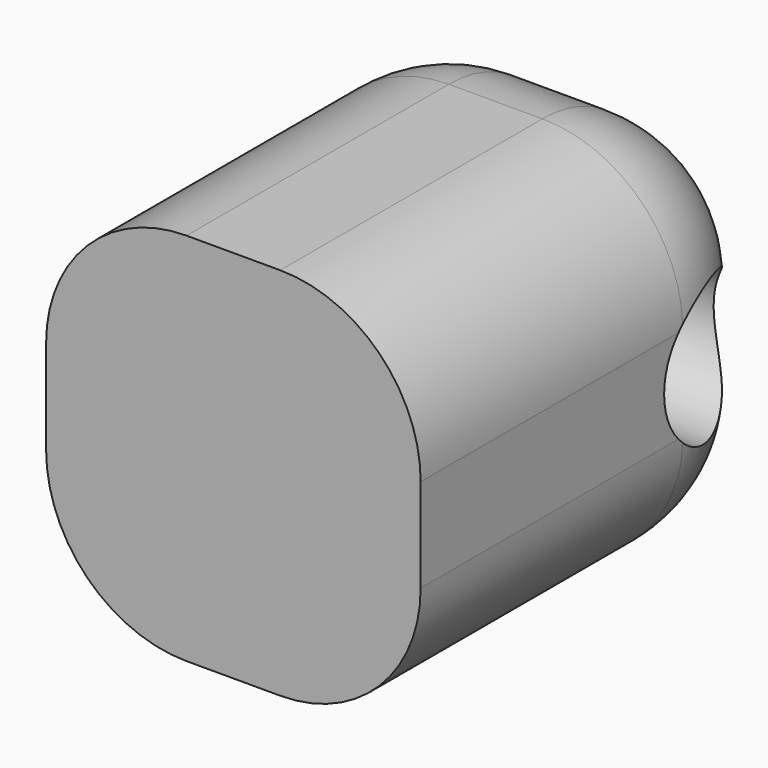
from build123d import *

# Parameters (mm, degrees)
F0_W         = 20
F0_H         = 20
F1_DEPTH     = 25
F2_R         = 3.75
F3_DEPTH     = 25
F4_R         = 7.5
F5_T1_DEPTH  = 36.25
F5_T3_DEPTH  = 5
F5_T6_ANGLE  = 90
F5_T8_ANGLE  = 90
F5_T10_ANGLE = 90
F5_T12_ANGLE = 90


# Not quite as in the source:
# - a fillet or chamfer that OpenCascade refuses, or shapes differently, is made with other operations: its cross-section is extruded or revolved along the edge and cut away or added


with BuildPart() as f1:
    # F0 (on Front) → F1 (new body)
    with BuildSketch(Plane.XZ):
        Rectangle(F0_W, F0_H)
    extrude(amount=F1_DEPTH)

    # F2 (on Right) → F3 (cut, symmetric)
    with BuildSketch(Plane.YZ):
        with Locations((-5, 0)):
            Circle(F2_R)
    extrude(amount=F3_DEPTH, both=True, mode=Mode.SUBTRACT)

    # F4
    f4_edges = [f1.edges().sort_by_distance(p)[0] for p in [
        (0, 0, 10),
        (0, 0, -10),
    ]]
    fillet(f4_edges, radius=F4_R)

    # F5: fillet of radius 7.5 on 8 edges, made by hand

    # F5_s2 → F5_t1 (cut)
    with BuildSketch(Plane.XZ.offset(7.5)):
        with BuildLine():
            ThreePointArc((-10, 2.5), (-7.8033008589, 7.8033008589), (-2.5, 10))
            Line((-2.5, 10), (-10, 10))
            Line((-10, 10), (-10, 2.5))
        make_face()
        with BuildLine():
            ThreePointArc((10, 2.5), (7.8033008589, 7.8033008589), (2.5, 10))
            Line((2.5, 10), (10, 10))
            Line((10, 10), (10, 2.5))
        make_face()
        with BuildLine():
            ThreePointArc((-2.5, -10), (-7.8033008589, -7.8033008589), (-10, -2.5))
            Line((-10, -2.5), (-10, -10))
            Line((-10, -10), (-2.5, -10))
        make_face()
        with BuildLine():
            ThreePointArc((2.5, -10), (7.8033008589, -7.8033008589), (10, -2.5))
            Line((10, -2.5), (10, -10))
            Line((10, -10), (2.5, -10))
        make_face()
    extrude(amount=F5_T1_DEPTH, mode=Mode.SUBTRACT)

    # F5_s4 → F5_t3 (cut)
    with BuildSketch(Plane.XY.offset(-2.5)):
        with BuildLine():
            ThreePointArc((10, -7.5), (7.8033008589, -2.1966991411), (2.5, 0))
            Line((2.5, 0), (10, 0))
            Line((10, 0), (10, -7.5))
        make_face()
        with BuildLine():
            ThreePointArc((-10, -7.5), (-7.8033008589, -2.1966991411), (-2.5, 0))
            Line((-2.5, 0), (-10, 0))
            Line((-10, 0), (-10, -7.5))
        make_face()
    extrude(amount=F5_T3_DEPTH, mode=Mode.SUBTRACT)

    # F5_s5 → F5_t6 (revolve, cut)
    with BuildSketch(Plane.XY.offset(2.5)):
        with BuildLine():
            ThreePointArc((-10, -7.5), (-7.8033008589, -2.1966991411), (-2.5, 0))
            Line((-2.5, 0), (-10, 0))
            Line((-10, 0), (-10, -7.5))
        make_face()
    revolve(axis=Axis((-10, -7.5, 2.5), (1, 0, 0)), revolution_arc=F5_T6_ANGLE, mode=Mode.SUBTRACT)

    # F5_s7 → F5_t8 (revolve, cut)
    with BuildSketch(Plane.XZ.offset(7.5)):
        with BuildLine():
            ThreePointArc((-10, -2.5), (-7.8033008589, -7.8033008589), (-2.5, -10))
            Line((-2.5, -10), (-10, -10))
            Line((-10, -10), (-10, -2.5))
        make_face()
    revolve(axis=Axis((-10, -7.5, -2.5), (1, 0, 0)), revolution_arc=F5_T8_ANGLE, mode=Mode.SUBTRACT)

    # F5_s9 → F5_t10 (revolve, cut)
    with BuildSketch(Plane.XZ.offset(7.5)):
        with BuildLine():
            ThreePointArc((2.5, -10), (7.8033008589, -7.8033008589), (10, -2.5))
            Line((10, -2.5), (10, -10))
            Line((10, -10), (2.5, -10))
        make_face()
    revolve(axis=Axis((10, -7.5, -2.5), (1, 0, 0)), revolution_arc=F5_T10_ANGLE, mode=Mode.SUBTRACT)

    # F5_s11 → F5_t12 (revolve, cut)
    with BuildSketch(Plane.XY.offset(2.5)):
        with BuildLine():
            ThreePointArc((10, -7.5), (7.8033008589, -2.1966991411), (2.5, 0))
            Line((2.5, 0), (10, 0))
            Line((10, 0), (10, -7.5))
        make_face()
    revolve(axis=Axis((10, -7.5, 2.5), (1, 0, 0)), revolution_arc=F5_T12_ANGLE, mode=Mode.SUBTRACT)


solid = f1.part
